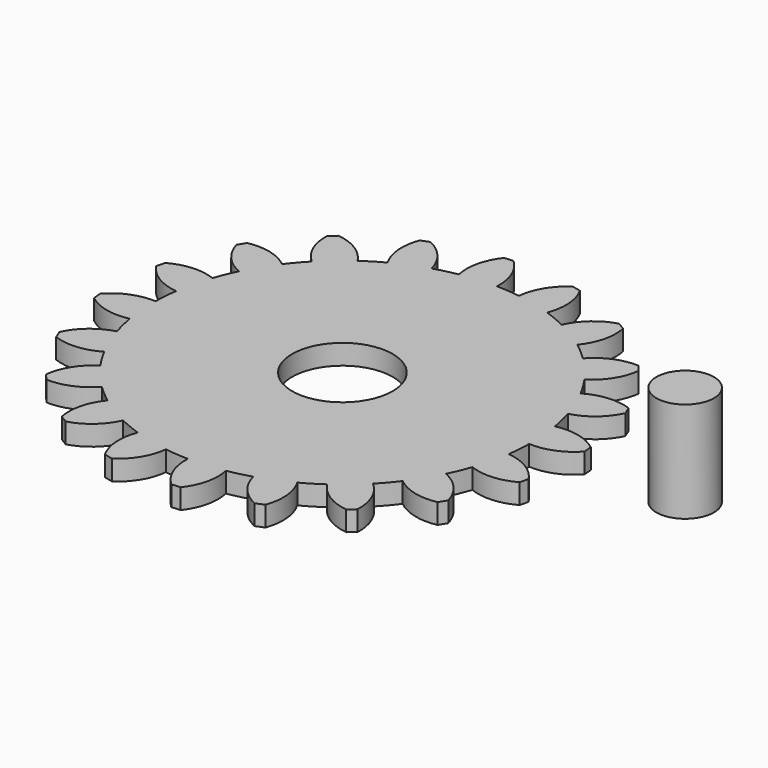
from build123d import *

# Parameters (mm, degrees)
F2_R     = 2.5
F3_DEPTH = 1
F4_R     = 1.4288855247
F5_DEPTH = 5


# Not quite as in the source:
# - a feature of the source that left no trace in its solid (it failed there, or was rolled back) is left out


with BuildPart() as f3:
    # F2 (on Top) → F3 (new body)
    with BuildSketch(Plane.XY):
        with BuildLine():
            ThreePointArc((-1.6229776334, 9.2680599554), (-0.7382287643, 9.3800858219), (0.1531520845, 9.4078443957))
            ThreePointArc((0.1531520845, 9.4078443957), (-0.0317997207, 10.5374998224), (-0.6817601701, 11.4797736507))
            Line((-0.6817601701, 11.4797736507), (-1.1224656787, 11.4450893749))
            ThreePointArc((-1.1224656787, 11.4450893749), (-1.6170199342, 10.4127402859), (-1.6229776334, 9.2680599554))
        make_face()
        with BuildLine():
            ThreePointArc((9.4078443957, -0.1531520845), (9.4087792756, -0.0765785786), (9.4090909091, 0))
            ThreePointArc((9.4090909091, 0), (9.3737668631, 0.8145468262), (9.2680599554, 1.6229776334))
            ThreePointArc((9.2680599554, 1.6229776334), (9.1491169783, 2.1965086508), (8.9947183137, 2.7615275108))
            ThreePointArc((8.9947183137, 2.7615275108), (8.6928665104, 3.6007032045), (8.3129211438, 4.4075314852))
            ThreePointArc((8.3129211438, 4.4075314852), (8.0225688191, 4.9162364953), (7.7011265332, 5.4058895526))
            ThreePointArc((7.7011265332, 5.4058895526), (7.1547288581, 6.1107157275), (6.5440556911, 6.7606454461))
            ThreePointArc((6.5440556911, 6.7606454461), (6.1107157275, 7.1547288581), (5.6536948308, 7.52108546))
            ThreePointArc((5.6536948308, 7.52108546), (4.9162364953, 8.0225688191), (4.1346124722, 8.4519803265))
            ThreePointArc((4.1346124722, 8.4519803265), (3.6007032045, 8.6928665104), (3.0528400867, 8.90006512))
            ThreePointArc((3.0528400867, 8.90006512), (2.1965086508, 9.1491169783), (1.320444577, 9.3159764842))
            ThreePointArc((1.320444577, 9.3159764842), (0.7382287643, 9.3800858219), (0.1531520845, 9.4078443957))
            ThreePointArc((0.1531520845, 9.4078443957), (-0.7382287643, 9.3800858219), (-1.6229776334, 9.2680599554))
            ThreePointArc((-1.6229776334, 9.2680599554), (-2.1965086508, 9.1491169783), (-2.7615275108, 8.9947183137))
            ThreePointArc((-2.7615275108, 8.9947183137), (-3.6007032045, 8.6928665104), (-4.4075314852, 8.3129211438))
            ThreePointArc((-4.4075314852, 8.3129211438), (-4.9162364953, 8.0225688191), (-5.4058895526, 7.7011265332))
            ThreePointArc((-5.4058895526, 7.7011265332), (-6.1107157275, 7.1547288581), (-6.7606454461, 6.5440556911))
            ThreePointArc((-6.7606454461, 6.5440556911), (-7.1547288581, 6.1107157275), (-7.52108546, 5.6536948308))
            ThreePointArc((-7.52108546, 5.6536948308), (-8.0225688191, 4.9162364953), (-8.4519803265, 4.1346124722))
            ThreePointArc((-8.4519803265, 4.1346124722), (-8.6928665104, 3.6007032045), (-8.90006512, 3.0528400867))
            ThreePointArc((-8.90006512, 3.0528400867), (-9.1491169783, 2.1965086508), (-9.3159764842, 1.320444577))
            ThreePointArc((-9.3159764842, 1.320444577), (-9.3800858219, 0.7382287643), (-9.4078443957, 0.1531520845))
            ThreePointArc((-9.4078443957, 0.1531520845), (-9.3800858219, -0.7382287643), (-9.2680599554, -1.6229776334))
            ThreePointArc((-9.2680599554, -1.6229776334), (-9.1491169783, -2.1965086508), (-8.9947183137, -2.7615275108))
            ThreePointArc((-8.9947183137, -2.7615275108), (-8.6928665104, -3.6007032045), (-8.3129211438, -4.4075314852))
            ThreePointArc((-8.3129211438, -4.4075314852), (-8.0225688191, -4.9162364953), (-7.7011265332, -5.4058895526))
            ThreePointArc((-7.7011265332, -5.4058895526), (-7.1547288581, -6.1107157275), (-6.5440556911, -6.7606454461))
            ThreePointArc((-6.5440556911, -6.7606454461), (-6.1107157275, -7.1547288581), (-5.6536948308, -7.52108546))
            ThreePointArc((-5.6536948308, -7.52108546), (-4.9162364953, -8.0225688191), (-4.1346124722, -8.4519803265))
            ThreePointArc((-4.1346124722, -8.4519803265), (-3.6007032045, -8.6928665104), (-3.0528400867, -8.90006512))
            ThreePointArc((-3.0528400867, -8.90006512), (-2.1965086508, -9.1491169783), (-1.320444577, -9.3159764842))
            ThreePointArc((-1.320444577, -9.3159764842), (-0.7382287643, -9.3800858219), (-0.1531520845, -9.4078443957))
            ThreePointArc((-0.1531520845, -9.4078443957), (0.7382287643, -9.3800858219), (1.6229776334, -9.2680599554))
            ThreePointArc((1.6229776334, -9.2680599554), (2.1965086508, -9.1491169783), (2.7615275108, -8.9947183137))
            ThreePointArc((2.7615275108, -8.9947183137), (3.6007032045, -8.6928665104), (4.4075314852, -8.3129211438))
            ThreePointArc((4.4075314852, -8.3129211438), (4.9162364953, -8.0225688191), (5.4058895526, -7.7011265332))
            ThreePointArc((5.4058895526, -7.7011265332), (6.1107157275, -7.1547288581), (6.7606454461, -6.5440556911))
            ThreePointArc((6.7606454461, -6.5440556911), (7.1547288581, -6.1107157275), (7.52108546, -5.6536948308))
            ThreePointArc((7.52108546, -5.6536948308), (8.0225688191, -4.9162364953), (8.4519803265, -4.1346124722))
            ThreePointArc((8.4519803265, -4.1346124722), (8.6928665104, -3.6007032045), (8.90006512, -3.0528400867))
            ThreePointArc((8.90006512, -3.0528400867), (9.1491169783, -2.1965086508), (9.3159764842, -1.320444577))
            ThreePointArc((9.3159764842, -1.320444577), (9.3800858219, -0.7382287643), (9.4078443957, -0.1531520845))
        make_face()
        Circle(F2_R, mode=Mode.SUBTRACT)
        with BuildLine():
            ThreePointArc((-4.4075314852, 8.3129211438), (-3.6007032045, 8.6928665104), (-2.7615275108, 8.9947183137))
            ThreePointArc((-2.7615275108, 8.9947183137), (-3.286509855, 10.0119312174), (-4.195837602, 10.7072380574))
            Line((-4.195837602, 10.7072380574), (-4.604255417, 10.5380658593))
            ThreePointArc((-4.604255417, 10.5380658593), (-4.7555910517, 9.4034178615), (-4.4075314852, 8.3129211438))
        make_face()
        with BuildLine():
            ThreePointArc((-6.7606454461, 6.5440556911), (-6.1107157275, 7.1547288581), (-5.4058895526, 7.7011265332))
            ThreePointArc((-5.4058895526, 7.7011265332), (-6.2195135061, 8.5063250277), (-7.2991972152, 8.8866034014))
            Line((-7.2991972152, 8.8866034014), (-7.6353485554, 8.5995030343))
            ThreePointArc((-7.6353485554, 8.5995030343), (-7.428651783, 7.4736233793), (-6.7606454461, 6.5440556911))
        make_face()
        with BuildLine():
            ThreePointArc((-8.4519803265, 4.1346124722), (-8.0225688191, 4.9162364953), (-7.52108546, 5.6536948308))
            ThreePointArc((-7.52108546, 5.6536948308), (-8.5437078414, 6.1680604771), (-9.6880605486, 6.1960860878))
            Line((-9.6880605486, 6.1960860878), (-9.9190405786, 5.8191609361))
            ThreePointArc((-9.9190405786, 5.8191609361), (-9.3745443193, 4.812258569), (-8.4519803265, 4.1346124722))
        make_face()
        with BuildLine():
            ThreePointArc((-9.3159764842, 1.320444577), (-9.1491169783, 2.1965086508), (-8.90006512, 3.0528400867))
            ThreePointArc((-8.90006512, 3.0528400867), (-10.0315845257, 3.2260231917), (-11.1285890147, 2.8990526973))
            Line((-11.1285890147, 2.8990526973), (-11.2317877999, 2.469198821))
            ThreePointArc((-11.2317877999, 2.469198821), (-10.4027911413, 1.679836361), (-9.3159764842, 1.320444577))
        make_face()
        with BuildLine():
            ThreePointArc((-9.2680599554, -1.6229776334), (-9.3800858219, -0.7382287643), (-9.4078443957, 0.1531520845))
            ThreePointArc((-9.4078443957, 0.1531520845), (-10.5374998224, -0.0317997207), (-11.4797736507, -0.6817601701))
            Line((-11.4797736507, -0.6817601701), (-11.4450893749, -1.1224656787))
            ThreePointArc((-11.4450893749, -1.1224656787), (-10.4127402859, -1.6170199342), (-9.2680599554, -1.6229776334))
        make_face()
        with BuildLine():
            ThreePointArc((-10.5380658593, -4.604255417), (-9.4034178615, -4.7555910517), (-8.3129211438, -4.4075314852))
            ThreePointArc((-8.3129211438, -4.4075314852), (-8.6928665104, -3.6007032045), (-8.9947183137, -2.7615275108))
            ThreePointArc((-8.9947183137, -2.7615275108), (-10.0119312174, -3.286509855), (-10.7072380574, -4.195837602))
            Line((-10.7072380574, -4.195837602), (-10.5380658593, -4.604255417))
        make_face()
        with BuildLine():
            ThreePointArc((-8.5995030343, -7.6353485554), (-7.4736233793, -7.428651783), (-6.5440556911, -6.7606454461))
            ThreePointArc((-6.5440556911, -6.7606454461), (-7.1547288581, -6.1107157275), (-7.7011265332, -5.4058895526))
            ThreePointArc((-7.7011265332, -5.4058895526), (-8.5063250277, -6.2195135061), (-8.8866034014, -7.2991972152))
            Line((-8.8866034014, -7.2991972152), (-8.5995030343, -7.6353485554))
        make_face()
        with BuildLine():
            ThreePointArc((-5.8191609361, -9.9190405786), (-4.812258569, -9.3745443193), (-4.1346124722, -8.4519803265))
            ThreePointArc((-4.1346124722, -8.4519803265), (-4.9162364953, -8.0225688191), (-5.6536948308, -7.52108546))
            ThreePointArc((-5.6536948308, -7.52108546), (-6.1680604771, -8.5437078414), (-6.1960860878, -9.6880605486))
            Line((-6.1960860878, -9.6880605486), (-5.8191609361, -9.9190405786))
        make_face()
        with BuildLine():
            ThreePointArc((-2.469198821, -11.2317877999), (-1.679836361, -10.4027911413), (-1.320444577, -9.3159764842))
            ThreePointArc((-1.320444577, -9.3159764842), (-2.1965086508, -9.1491169783), (-3.0528400867, -8.90006512))
            ThreePointArc((-3.0528400867, -8.90006512), (-3.2260231917, -10.0315845257), (-2.8990526973, -11.1285890147))
            Line((-2.8990526973, -11.1285890147), (-2.469198821, -11.2317877999))
        make_face()
        with BuildLine():
            ThreePointArc((1.1224656787, -11.4450893749), (1.6170199342, -10.4127402859), (1.6229776334, -9.2680599554))
            ThreePointArc((1.6229776334, -9.2680599554), (0.7382287643, -9.3800858219), (-0.1531520845, -9.4078443957))
            ThreePointArc((-0.1531520845, -9.4078443957), (0.0317997207, -10.5374998224), (0.6817601701, -11.4797736507))
            Line((0.6817601701, -11.4797736507), (1.1224656787, -11.4450893749))
        make_face()
        with BuildLine():
            ThreePointArc((4.604255417, -10.5380658593), (4.7555910517, -9.4034178615), (4.4075314852, -8.3129211438))
            ThreePointArc((4.4075314852, -8.3129211438), (3.6007032045, -8.6928665104), (2.7615275108, -8.9947183137))
            ThreePointArc((2.7615275108, -8.9947183137), (3.286509855, -10.0119312174), (4.195837602, -10.7072380574))
            Line((4.195837602, -10.7072380574), (4.604255417, -10.5380658593))
        make_face()
        with BuildLine():
            ThreePointArc((7.6353485554, -8.5995030343), (7.428651783, -7.4736233793), (6.7606454461, -6.5440556911))
            ThreePointArc((6.7606454461, -6.5440556911), (6.1107157275, -7.1547288581), (5.4058895526, -7.7011265332))
            ThreePointArc((5.4058895526, -7.7011265332), (6.2195135061, -8.5063250277), (7.2991972152, -8.8866034014))
            Line((7.2991972152, -8.8866034014), (7.6353485554, -8.5995030343))
        make_face()
        with BuildLine():
            ThreePointArc((9.9190405786, -5.8191609361), (9.3745443193, -4.812258569), (8.4519803265, -4.1346124722))
            ThreePointArc((8.4519803265, -4.1346124722), (8.0225688191, -4.9162364953), (7.52108546, -5.6536948308))
            ThreePointArc((7.52108546, -5.6536948308), (8.5437078414, -6.1680604771), (9.6880605486, -6.1960860878))
            Line((9.6880605486, -6.1960860878), (9.9190405786, -5.8191609361))
        make_face()
        with BuildLine():
            ThreePointArc((11.2317877999, -2.469198821), (10.4027911413, -1.679836361), (9.3159764842, -1.320444577))
            ThreePointArc((9.3159764842, -1.320444577), (9.1491169783, -2.1965086508), (8.90006512, -3.0528400867))
            ThreePointArc((8.90006512, -3.0528400867), (10.0315845257, -3.2260231917), (11.1285890147, -2.8990526973))
            Line((11.1285890147, -2.8990526973), (11.2317877999, -2.469198821))
        make_face()
        with BuildLine():
            ThreePointArc((9.2680599554, 1.6229776334), (9.3737668631, 0.8145468262), (9.4090909091, 0))
            ThreePointArc((9.4090909091, 0), (9.4087792756, -0.0765785786), (9.4078443957, -0.1531520845))
            ThreePointArc((9.4078443957, -0.1531520845), (10.5374998224, 0.0317997207), (11.4797736507, 0.6817601701))
            Line((11.4797736507, 0.6817601701), (11.4450893749, 1.1224656787))
            ThreePointArc((11.4450893749, 1.1224656787), (10.4127402859, 1.6170199342), (9.2680599554, 1.6229776334))
        make_face()
        with BuildLine():
            ThreePointArc((8.3129211438, 4.4075314852), (8.6928665104, 3.6007032045), (8.9947183137, 2.7615275108))
            ThreePointArc((8.9947183137, 2.7615275108), (10.0119312174, 3.286509855), (10.7072380574, 4.195837602))
            Line((10.7072380574, 4.195837602), (10.5380658593, 4.604255417))
            ThreePointArc((10.5380658593, 4.604255417), (9.4034178615, 4.7555910517), (8.3129211438, 4.4075314852))
        make_face()
        with BuildLine():
            ThreePointArc((6.5440556911, 6.7606454461), (7.1547288581, 6.1107157275), (7.7011265332, 5.4058895526))
            ThreePointArc((7.7011265332, 5.4058895526), (8.5063250277, 6.2195135061), (8.8866034014, 7.2991972152))
            Line((8.8866034014, 7.2991972152), (8.5995030343, 7.6353485554))
            ThreePointArc((8.5995030343, 7.6353485554), (7.4736233793, 7.428651783), (6.5440556911, 6.7606454461))
        make_face()
        with BuildLine():
            ThreePointArc((4.1346124722, 8.4519803265), (4.9162364953, 8.0225688191), (5.6536948308, 7.52108546))
            ThreePointArc((5.6536948308, 7.52108546), (6.1680604771, 8.5437078414), (6.1960860878, 9.6880605486))
            Line((6.1960860878, 9.6880605486), (5.8191609361, 9.9190405786))
            ThreePointArc((5.8191609361, 9.9190405786), (4.812258569, 9.3745443193), (4.1346124722, 8.4519803265))
        make_face()
        with BuildLine():
            ThreePointArc((1.320444577, 9.3159764842), (2.1965086508, 9.1491169783), (3.0528400867, 8.90006512))
            ThreePointArc((3.0528400867, 8.90006512), (3.2260231917, 10.0315845257), (2.8990526973, 11.1285890147))
            Line((2.8990526973, 11.1285890147), (2.469198821, 11.2317877999))
            ThreePointArc((2.469198821, 11.2317877999), (1.679836361, 10.4027911413), (1.320444577, 9.3159764842))
        make_face()
    extrude(amount=F3_DEPTH)


with BuildPart() as f5:
    # F4 (on Top) → F5 (new body)
    with BuildSketch(Plane.XY):
        with Locations((15.9734264016, 1.325807767)):
            Circle(F4_R)
    extrude(amount=F5_DEPTH)


solid = Compound([f3.part, f5.part])
